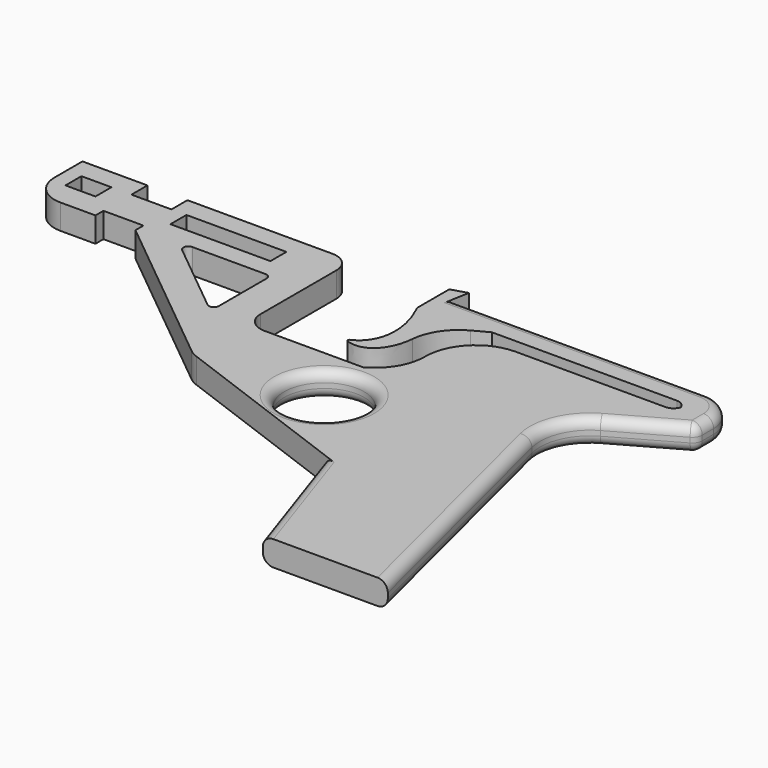
from build123d import *

# Parameters (mm, degrees)
F0_W     = 7.62
F0_H     = 5.08
F0_W_2   = 25.4
F0_R     = 10.16
F1_DEPTH = 6.35
F2_R     = 2.54


with BuildPart() as f1:
    # F0 (on Top) → F1 (new body)
    with BuildSketch(Plane.XY):
        with BuildLine():
            Line((-31.6706262529, -6.5881243579), (15.2908454792, -6.5881243579))
            ThreePointArc((15.2908454792, -6.5881243579), (16.7968803502, -7.0827737847), (17.7163331065, -8.374062179))
            ThreePointArc((17.7163331065, -8.374062179), (16.7968803502, -9.6653505732), (15.2908454792, -10.16))
            Line((15.2908454792, -10.16), (-22.8091545208, -10.16))
            ThreePointArc((-22.8091545208, -10.16), (-31.7894106419, -13.8797438789), (-35.5091545208, -22.86))
            Line((-35.5091545208, -22.86), (-35.5091545208, -23.067451765))
            ThreePointArc((-35.5091545208, -23.067451765), (-37.3281393906, -29.6167654494), (-42.2640379439, -34.29))
            Line((-42.2640379439, -34.29), (-67.31, -34.29))
            ThreePointArc((-67.31, -34.29), (-70.9021024484, -32.8021024484), (-72.39, -29.21))
            Line((-72.39, -29.21), (-72.39, -5.08))
            ThreePointArc((-72.39, -5.08), (-73.8778975516, -1.4878975516), (-77.47, 0))
            Line((-77.47, 0), (-114.3, 0))
            Line((-114.3, 0), (-114.3, -5.08))
            Line((-114.3, -5.08), (-124.46, -5.08))
            Line((-124.46, -5.08), (-124.46, 0))
            Line((-124.46, 0), (-140.97, 0))
            Line((-140.97, 0), (-140.97, -8.89))
            ThreePointArc((-140.97, -8.89), (-138.7381536726, -14.2781536726), (-133.35, -16.51))
            Line((-133.35, -16.51), (-124.46, -16.51))
            Line((-124.46, -16.51), (-124.46, -13.97))
            Line((-124.46, -13.97), (-114.3, -13.97))
            Line((-114.3, -13.97), (-114.3, -16.51))
            Line((-114.3, -16.51), (-73.1955929906, -50.0475420508))
            ThreePointArc((-73.1955929906, -50.0475420508), (-72.1633213981, -50.756926583), (-71.0287858488, -51.2876243715))
            Line((-71.0287858488, -51.2876243715), (-24.3288669735, -68.6128414369))
            Line((-24.3288669735, -68.6128414369), (-12.7, -103.0557602644))
            Line((-12.7, -103.0557602644), (19.05, -103.0557602644))
            Line((19.05, -103.0557602644), (2.3547967276, -36.4372610145))
            ThreePointArc((2.3547967276, -36.4372610145), (3.0065319132, -28.3336286948), (8.4393105622, -22.2856098724))
            Line((8.4393105622, -22.2856098724), (24.1577511408, -13.4286290107))
            ThreePointArc((24.1577511408, -13.4286290107), (25.1038731102, -12.4972467832), (25.4508454792, -11.2157516369))
            Line((25.4508454792, -11.2157516369), (25.4508454792, -7.62))
            ThreePointArc((25.4508454792, -7.62), (23.2189991518, -2.2318463274), (17.8308454792, 0))
            Line((17.8308454792, 0), (12.0385419577, 0))
            Line((12.0385419577, 0), (-46.4872904122, 0))
            Line((-46.4872904122, 0), (-45.8256908553, 3.752117539))
            Line((-45.8256908553, 3.752117539), (-49.8210415244, 2.54))
            Line((-49.8210415244, 2.54), (-49.8210415244, 0))
            Line((-49.8210415244, 0), (-49.8210415244, -7.5935418718))
            add(Edge.make_bspline(
                [(-49.8210415244, -7.5935418718), (-44.485431179, -18.5982405148), (-47.5559489311, -24.9495477887), (-51.5999285014, -26.6474626741)],
                knots=[0, 0, 0, 0, 17.7354547772, 17.7354547772, 17.7354547772, 17.7354547772], degree=3))
            ThreePointArc((-51.5999285014, -26.6474626741), (-51.8920952454, -27.1191706564), (-51.5419420272, -27.5495920205))
            add(Edge.make_bspline(
                [(-42.1931219537, -18.7228273079), (-42.6397200116, -23.7693324215), (-45.6204470158, -29.1828876463), (-51.5419420272, -27.5495920205)],
                knots=[5.2109253832, 5.2109253832, 5.2109253832, 5.2109253832, 16.5043202027, 16.5043202027, 16.5043202027, 16.5043202027], degree=3))
            ThreePointArc((-42.1931219537, -18.7228273079), (-40.130905812, -12.8297269732), (-35.5096463796, -8.6314739761))
            Line((-35.5096463796, -8.6314739761), (-31.6706262529, -6.5881243579))
        make_face()
        with BuildLine():
            Line((-83.0959535938, -32.5987200656), (-101.7744590691, -17.3587200656))
            ThreePointArc((-101.7744590691, -17.3587200656), (-102.1679568897, -15.9485577312), (-100.9715862663, -15.1047001153))
            Line((-100.9715862663, -15.1047001153), (-82.2930807911, -15.1047001153))
            ThreePointArc((-82.2930807911, -15.1047001153), (-81.3950551789, -15.4766745032), (-81.0230807911, -16.3747001153))
            Line((-81.0230807911, -16.3747001153), (-81.0230807911, -31.6147001153))
            ThreePointArc((-81.0230807911, -31.6147001153), (-81.74844718, -32.7619900655), (-83.0959535938, -32.5987200656))
        make_face(mode=Mode.SUBTRACT)
        with Locations((-133.35, -7.62)):
            Rectangle(F0_W, F0_H, mode=Mode.SUBTRACT)
        with Locations((-97.79, -7.62)):
            Rectangle(F0_W_2, F0_H, mode=Mode.SUBTRACT)
        with Locations((-40.8155657351, -48.4425649047)):
            Circle(F0_R, mode=Mode.SUBTRACT)
        with BuildLine():
            ThreePointArc((17.8308454792, -9.1281243579), (17.8020542094, -8.7467705677), (17.7163331065, -8.374062179))
            ThreePointArc((17.7163331065, -8.374062179), (17.8020542094, -8.0013537902), (17.8308454792, -7.62))
            Line((17.8308454792, -7.62), (17.8308454792, -9.1281243579))
        make_face(mode=Mode.SUBTRACT)
        with BuildLine():
            ThreePointArc((17.8308454792, -7.62), (17.8020542094, -8.0013537902), (17.7163331065, -8.374062179))
            ThreePointArc((17.7163331065, -8.374062179), (17.8020542094, -8.7467705677), (17.8308454792, -9.1281243579))
            Line((17.8308454792, -9.1281243579), (17.8308454792, -7.62))
        make_face()
    extrude(amount=F1_DEPTH)

    # F2
    f2_edges = [f1.edges().sort_by_distance(p)[0] for p in [
        (-18.514433, -85.834301, 6.35),
        (-18.514433, -85.834301, 0),
        (-50.975566, -48.442565, 6.35),
        (-50.975566, -48.442565, 0),
        (10.702398, -69.746511, 6.35),
        (10.702398, -69.746511, 0),
        (3.006532, -28.333629, 0),
        (3.006532, -28.333629, 6.35),
        (16.298531, -17.857119, 0),
        (16.298531, -17.857119, 6.35),
        (25.103873, -12.497247, 0),
        (25.103873, -12.497247, 6.35),
        (25.450845, -9.417876, 0),
        (25.450845, -9.417876, 6.35),
        (23.218999, -2.231846, 0),
        (23.218999, -2.231846, 6.35),
        (-14.328222, 0, 0),
        (-14.328222, 0, 6.35),
    ]]
    fillet(f2_edges, radius=F2_R)


solid = f1.part
